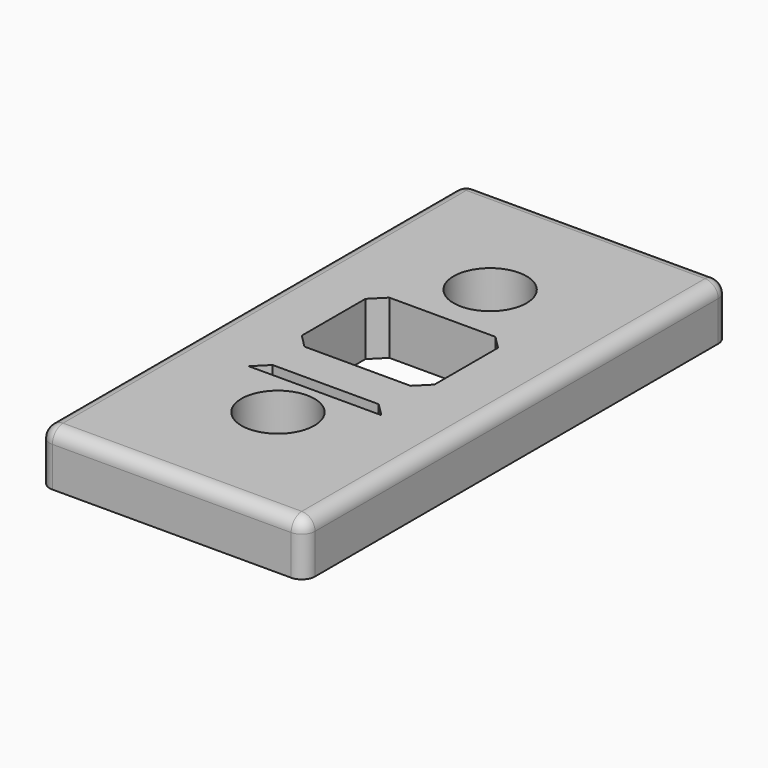
from build123d import *

# Parameters (mm, degrees)
F5_W     = 20
F5_H     = 40
F6_DEPTH = 4
F1_D     = 5.5
F2_R     = 1
F7_W     = 10
F7_H     = 1
F8_DEPTH = 25
F3_R     = 1
F4_SIZE  = 0.99999


# Not quite as in the source:
# - a fillet or chamfer is up to 0.001 mm smaller than in the source, because OpenCascade refuses the exact size
# - a feature names something its author has since deleted; it is built from what else it names


with BuildPart() as f6:
    # F5 (on Top) → F6 (new body)
    with BuildSketch(Plane.XY):
        Rectangle(F5_W, F5_H)
    extrude(amount=F6_DEPTH)

    # F1 (through all)
    with Locations(Plane.XY.offset(4)):
        with Locations((0, 10), (0, -10)):
            Hole(F1_D / 2)

    # F2
    f2_edges = [f6.edges().sort_by_distance(p)[0] for p in [
        (-10, -20, 2),
        (10, -20, 2),
        (-10, 20, 2),
        (10, 20, 2),
    ]]
    fillet(f2_edges, radius=F2_R)

    # F7 (on face) → F8 (cut)
    with BuildSketch(Plane.XY.offset(4)):
        Polygon((-5, -2.5), (5, -2.5), (5, 2.5), (5, 5.5), (-5, 5.5), (-5, 2.5), align=None)
        with Locations((0, -6)):
            Rectangle(F7_W, F7_H)
    extrude(amount=-F8_DEPTH, mode=Mode.SUBTRACT)

    # F3
    f3_edges = [f6.edges().sort_by_distance(p)[0] for p in [
        (0, -20, 4),
        (10, 0, 4),
        (0, 20, 4),
        (-10, 0, 4),
    ]]
    fillet(f3_edges, radius=F3_R)

    # F4 (size 1 in the source; OpenCascade refuses exactly that, so slightly less here)
    f4_edges = [f6.edges().sort_by_distance(p)[0] for p in [
        (-5, -5.5, 2),
        (5, -5.5, 2),
        (5, 5.5, 2),
        (-5, 5.5, 2),
        (-5, -2.5, 2),
        (5, -2.5, 2),
    ]]
    chamfer(f4_edges, length=F4_SIZE)


solid = f6.part
